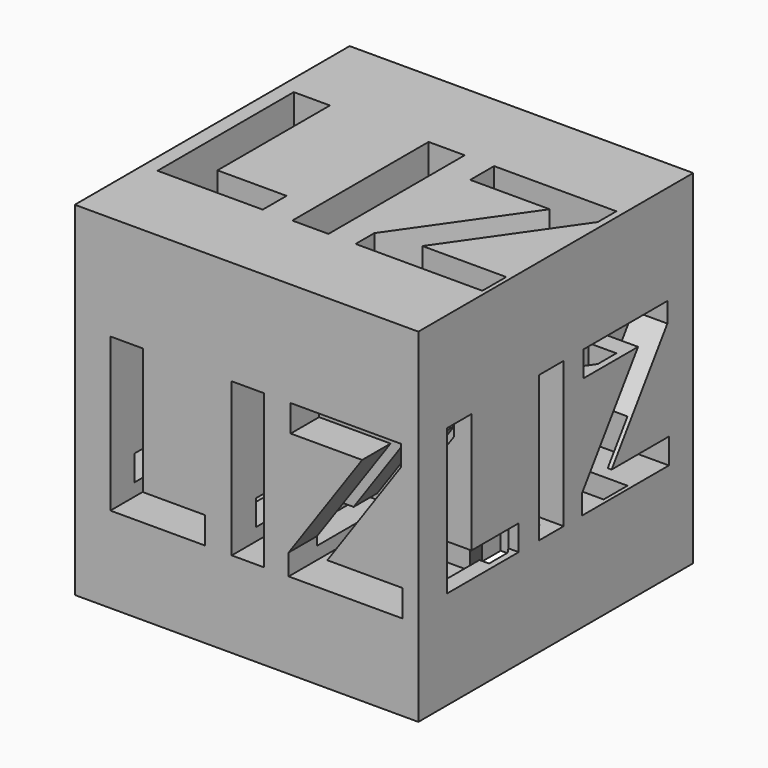
from build123d import *

# Parameters (mm, degrees)
F0_W          = 50.8
F0_H          = 50.8
F1_DEPTH      = 50.8
F2_TEXT_SIZE  = 30.1564464599
F3_DEPTH      = 25.4
F4_TEXT_SIZE  = 31.75
F5_DEPTH      = 25.4
F6_TEXT_SIZE  = 30.6590539009
F7_DEPTH      = 25.4
F8_TEXT_SIZE  = 30.1564464599
F9_DEPTH      = 25.4
F10_TEXT_SIZE = 35.2777777778
F11_DEPTH     = 25.4
F12_TEXT_SIZE = 35.2777777778
F13_DEPTH     = 25.4


# Not quite as in the source:
# - Text() gives the source's letters only with a copy of the font that has no kerning and outlines rounded to 1/6400 em; it was checked with that copy


with BuildPart() as f1:
    # F0 (on Front) → F1 (new body)
    with BuildSketch(Plane.XZ):
        Rectangle(F0_W, F0_H)
    extrude(amount=F1_DEPTH)

    # F2 (on face) → F3 (cut)
    with BuildSketch(Plane.YZ.offset(25.4)):
        with Locations((-48.26, -10.8414414511)):
            Text('LIZ', F2_TEXT_SIZE, font='Open Sans', font_style=FontStyle.BOLD, text_align=(TextAlign.LEFT, TextAlign.BOTTOM))
    extrude(amount=-F3_DEPTH, mode=Mode.SUBTRACT)

    # F4 (on face) → F5 (cut)
    with BuildSketch(Plane.XZ.offset(50.8)):
        with Locations((-22.987, -12.7)):
            Text('LIZ', F4_TEXT_SIZE, font='Open Sans', font_style=FontStyle.BOLD, text_align=(TextAlign.LEFT, TextAlign.BOTTOM))
    extrude(amount=-F5_DEPTH, mode=Mode.SUBTRACT)

    # F6 (on face) → F7 (cut)
    with BuildSketch(Plane(origin=(0, 0, 0), x_dir=(-1, 0, 0), z_dir=(0, 1, 0))):
        with Locations((-23.1037839443, -10.4469084192)):
            Text('LIZ', F6_TEXT_SIZE, font='Open Sans', font_style=FontStyle.BOLD, text_align=(TextAlign.LEFT, TextAlign.BOTTOM))
    extrude(amount=-F7_DEPTH, mode=Mode.SUBTRACT)

    # F8 (on face) → F9 (cut)
    with BuildSketch(Plane(origin=(-25.4, 0, 0), x_dir=(0, -1, 0), z_dir=(-1, 0, 0))):
        with Locations((2.54, -10.8414414511)):
            Text('LIZ', F8_TEXT_SIZE, font='Open Sans', font_style=FontStyle.BOLD, text_align=(TextAlign.LEFT, TextAlign.BOTTOM))
    extrude(amount=-F9_DEPTH, mode=Mode.SUBTRACT)

    # F10 (on face) → F11 (cut)
    with BuildSketch(Plane.XY.offset(25.4)):
        with Locations((-26.4166382588, -38.2010390776)):
            Text('LIZ', F10_TEXT_SIZE, font='Open Sans', font_style=FontStyle.BOLD, text_align=(TextAlign.LEFT, TextAlign.BOTTOM))
    extrude(amount=-F11_DEPTH, mode=Mode.SUBTRACT)

    # F12 (on face) → F13 (cut)
    with BuildSketch(Plane(origin=(0, 0, -25.4), x_dir=(1, 0, 0), z_dir=(0, 0, -1))):
        with Locations((-26.3696751107, 11.43)):
            Text('LIZ', F12_TEXT_SIZE, font='Open Sans', font_style=FontStyle.BOLD, text_align=(TextAlign.LEFT, TextAlign.BOTTOM))
    extrude(amount=-F13_DEPTH, mode=Mode.SUBTRACT)


solid = f1.part
